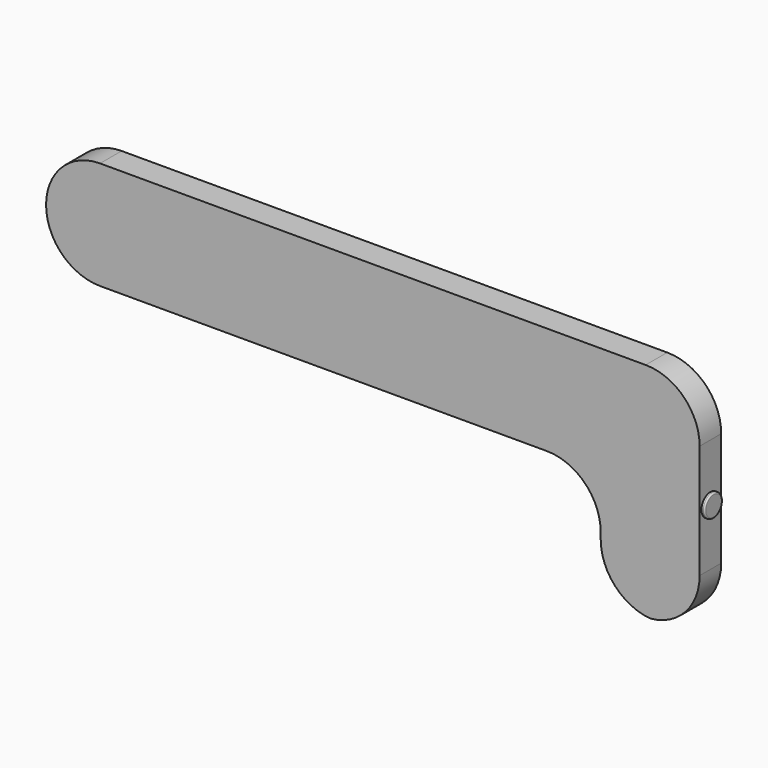
from build123d import *

# Parameters (mm, degrees)
F1_DEPTH    = 1.27
F2_T1_DEPTH = 2.54
F2_T3_DEPTH = 27.94
F3_R        = 5.07999
F4_R        = 1.0553612336
F5_DEPTH    = 0.3048
F6_R        = 0.127


# Not quite as in the source:
# - a fillet or chamfer that OpenCascade refuses, or shapes differently, is made with other operations: its cross-section is extruded or revolved along the edge and cut away or added
# - a fillet or chamfer is up to 0.001 mm smaller than in the source, because OpenCascade refuses the exact size


with BuildPart() as f1:
    # F0 (on Front) → F1 (new body, symmetric)
    with BuildSketch(Plane.XZ):
        Polygon((-46.589029785, 38.6476762999), (-46.589029785, 28.4876762999), (5.6178237253, 28.4876762999), (5.6178237253, 17.7632305365), (14.9303989669, 17.7632305365), (14.9303989669, 38.6476762999), align=None)
    extrude(amount=F1_DEPTH, both=True)

    # F2: fillet of radius 5.08 on 4 edges, made by hand

    # F2_s2 → F2_t1 (join)
    with BuildSketch(Plane.XZ.offset(-1.27)):
        with BuildLine():
            ThreePointArc((5.6178237253, 23.4076762999), (4.1299261737, 26.9997787484), (0.5378237253, 28.4876762999))
            Line((0.5378237253, 28.4876762999), (5.6178237253, 28.4876762999))
            Line((5.6178237253, 28.4876762999), (5.6178237253, 23.4076762999))
        make_face()
    extrude(amount=F2_T1_DEPTH)

    # F2_s4 → F2_t3 (cut)
    with BuildSketch(Plane.XZ.offset(-13.97)):
        with BuildLine():
            ThreePointArc((9.8503989669, 38.6476762999), (13.4425014153, 37.1597787484), (14.9303989669, 33.5676762999))
            Line((14.9303989669, 33.5676762999), (14.9303989669, 38.6476762999))
            Line((14.9303989669, 38.6476762999), (9.8503989669, 38.6476762999))
        make_face()
        with BuildLine():
            ThreePointArc((14.9303989669, 22.8432305365), (13.4425014153, 19.251128088), (9.8503989669, 17.7632305365))
            Line((9.8503989669, 17.7632305365), (14.9303989669, 17.7632305365))
            Line((14.9303989669, 17.7632305365), (14.9303989669, 22.8432305365))
        make_face()
        with BuildLine():
            ThreePointArc((5.6178237253, 22.8432305365), (7.1057212768, 19.251128088), (10.6978237253, 17.7632305365))
            Line((10.6978237253, 17.7632305365), (5.6178237253, 17.7632305365))
            Line((5.6178237253, 17.7632305365), (5.6178237253, 22.8432305365))
        make_face()
    extrude(amount=F2_T3_DEPTH, mode=Mode.SUBTRACT)

    # F3 (radius 5.08 in the source; OpenCascade refuses exactly that, so slightly less here)
    f3_edges = [f1.edges().sort_by_distance(p)[0] for p in [
        (-46.58903, 0, 38.647676),
        (-46.58903, 0, 28.487676),
    ]]
    fillet(f3_edges, radius=F3_R)


with BuildPart() as f5:
    # F4 (on face) → F5 (new body)
    with BuildSketch(Plane.YZ.offset(14.9303989669)):
        with Locations((0, 28.2054534182)):
            Circle(F4_R)
    extrude(amount=F5_DEPTH)

    # F6
    f6_edges = [f5.edges().sort_by_distance(p)[0] for p in [
        (15.235199, -1.055361, 28.205453),
    ]]
    fillet(f6_edges, radius=F6_R)


solid = Compound([f1.part, f5.part])
